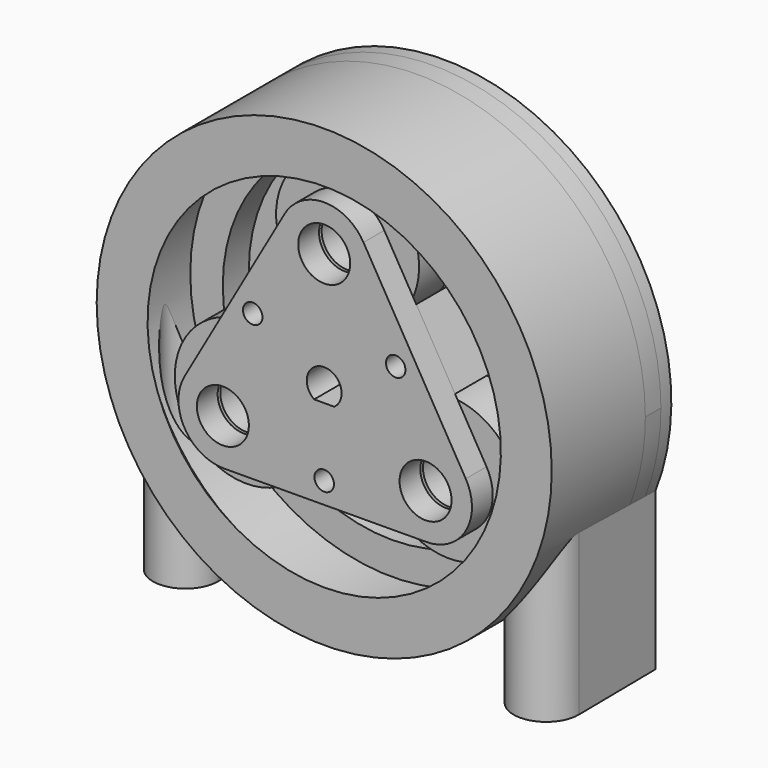
from build123d import *

# Parameters (mm, degrees)
F0_R      = 4
F1_DEPTH  = 4
F3_DEPTH  = 4
F4_R      = 1.5
F5_DEPTH  = 25.4
F7_R      = 35
F7_R_2    = 2.85
F7_R_3    = 4
F8_DEPTH  = 3
F9_R      = 35
F9_R_2    = 1.75
F9_R_3    = 4
F10_DEPTH = 2
F12_R     = 11
F12_R_2   = 4
F13_DEPTH = 7
F15_R     = 35
F15_R_2   = 31
F16_DEPTH = 18
F22_R     = 3.175
F23_DEPTH = 37
F24_R     = 31
F24_R_2   = 26
F25_DEPTH = 5


# Not quite as in the source:
# - after a boolean that leaves OpenCascade's solid faulty, fix() repairs it


with BuildPart() as f1:
    # F0 (on Front) → F1 (new body)
    with BuildSketch(Plane.XZ):
        with BuildLine():
            Line((21.7703811819, -5.3551862172), (6.0422815334, 21.5342373819))
            ThreePointArc((6.0422815334, 21.5342373819), (-0.039598589, 24.9998879957), (-6.0818801224, 21.4656506138))
            Line((-6.0818801224, 21.4656506138), (-21.504754228, -5.5999950346))
            ThreePointArc((-21.504754228, -5.5999950346), (-21.465155639, -12.5998830303), (-15.3832755166, -16.0655336441))
            Line((-15.3832755166, -16.0655336441), (15.7676982376, -15.8893115947))
            ThreePointArc((15.7676982376, -15.8893115947), (21.8099797709, -12.3550742128), (21.7703811819, -5.3551862172))
        make_face()
        with Locations((-15.5884572681, -9)):
            Circle(F0_R, mode=Mode.SUBTRACT)
        with Locations((15.5884572681, -9)):
            Circle(F0_R, mode=Mode.SUBTRACT)
        with Locations((0, 18)):
            Circle(F0_R, mode=Mode.SUBTRACT)
    extrude(amount=F1_DEPTH)

    # F2 (on face) → F3 (join)
    with BuildSketch(Plane.XZ.offset(4)):
        with BuildLine():
            ThreePointArc((-16.6300065653, 2.9547135081), (-5.1558488531, -3.0703556887), (-5.8500069609, -16.0116036406))
            Line((-5.8500069609, -16.0116036406), (5.8028816925, -15.9456828789))
            ThreePointArc((5.8028816925, -15.9456828789), (5.2509372213, -2.906094907), (16.9270942552, 2.9251017194))
            Line((16.9270942552, 2.9251017194), (10.9633508087, 13.1209694563))
            ThreePointArc((10.9633508087, 13.1209694563), (0.0678832955, 6.0001920074), (-10.9074492372, 12.9972456448))
            Line((-10.9074492372, 12.9972456448), (-16.6300065653, 2.9547135081))
        make_face()
        with BuildLine():
            ThreePointArc((-1.5447653543, -2.19), (0, 2.68), (1.5447653543, -2.19))
            Line((1.5447653543, -2.19), (-1.5447653543, -2.19))
        make_face(mode=Mode.SUBTRACT)
    extrude(amount=F3_DEPTH)

    # F4 (on Front) → F5 (cut)
    with BuildSketch(Plane.XZ):
        with Locations((0, -12.7)):
            Circle(F4_R)
        with Locations((10.9985226281, 6.35)):
            Circle(F4_R)
        with Locations((-10.9985226281, 6.35)):
            Circle(F4_R)
        with BuildLine():
            Line((-1.5447653543, -2.19), (1.5447653543, -2.19))
            ThreePointArc((1.5447653543, -2.19), (0, 2.68), (-1.5447653543, -2.19))
        make_face()
    extrude(amount=F5_DEPTH, mode=Mode.SUBTRACT)

    # F14: F1 across face


with BuildPart() as f8:
    # F7 (on offset) → F8 (new body)
    with BuildSketch(Plane.XZ.offset(-2)):
        Circle(F7_R)
        with Locations((-15.5, -15.5)):
            Circle(F7_R_2, mode=Mode.SUBTRACT)
        with Locations((15.5, -15.5)):
            Circle(F7_R_2, mode=Mode.SUBTRACT)
        with Locations((-15.5, 15.5)):
            Circle(F7_R_2, mode=Mode.SUBTRACT)
        Circle(F7_R_3, mode=Mode.SUBTRACT)
        with Locations((15.5, 15.5)):
            Circle(F7_R_2, mode=Mode.SUBTRACT)
    extrude(amount=-F8_DEPTH)

    # F9 (on face) → F10 (join)
    with BuildSketch(Plane(origin=(0, 5, 0), x_dir=(-1, 0, 0), z_dir=(0, 1, 0))):
        Circle(F9_R)
        with Locations((-15.5, -15.5)):
            Circle(F9_R_2, mode=Mode.SUBTRACT)
        with Locations((15.5, -15.5)):
            Circle(F9_R_2, mode=Mode.SUBTRACT)
        with Locations((-15.5, 15.5)):
            Circle(F9_R_2, mode=Mode.SUBTRACT)
        Circle(F9_R_3, mode=Mode.SUBTRACT)
        with Locations((15.5, 15.5)):
            Circle(F9_R_2, mode=Mode.SUBTRACT)
    extrude(amount=F10_DEPTH)

    # F15 (on face) → F16 (join)
    with BuildSketch(Plane.XZ.offset(-2)):
        Circle(F15_R)
        Circle(F15_R_2, mode=Mode.SUBTRACT)
    extrude(amount=F16_DEPTH)

    add(f8.part.fix(), mode=Mode.REPLACE)

    # F17 (on Right) → F18 (revolve)
    with BuildSketch(Plane.YZ):
        Polygon((-16, -32.175), (-11, -32.175), (-16, -27.175), align=None)
    revolve(axis=Axis((0, -8.0179562792, 0), (0, -1, 0)))

    # F20 (on offset) → F21 (join, up to the next surface of F8)
    with BuildSketch(Plane.XY.offset(-37)):
        with BuildLine():
            Line((-32.5682681475, 7), (-32.7496315906, -7.9393043761))
            ThreePointArc((-32.7496315906, -7.9393043761), (-27.7619081825, -12.9999858195), (-22.7501360182, -7.9631196072))
            Line((-22.7501360182, -7.9631196072), (-22.7501360182, 7))
            Line((-22.7501360182, 7), (-32.5682681475, 7))
        make_face()
        with BuildLine():
            ThreePointArc((22.7501360182, -7.9631196072), (27.7619081825, -12.9999858195), (32.7496315906, -7.9393043761))
            Line((32.7496315906, -7.9393043761), (32.5682681475, 7))
            Line((32.5682681475, 7), (22.7501360182, 7))
            Line((22.7501360182, 7), (22.7501360182, -7.9631196072))
        make_face()
    extrude(until=Until.NEXT)

    # F22 (on face) → F23 (cut)
    with BuildSketch(Plane(origin=(0, 0, -37), x_dir=(1, 0, 0), z_dir=(0, 0, -1))):
        with Locations((27.75, 8)):
            Circle(F22_R)
        with Locations((-27.75, 8)):
            Circle(F22_R)
    extrude(amount=-F23_DEPTH, mode=Mode.SUBTRACT)

    # F24 (on face) → F25 (join)
    with BuildSketch(Plane.XZ.offset(-2)):
        Circle(F24_R)
        Circle(F24_R_2, mode=Mode.SUBTRACT)
    extrude(amount=F25_DEPTH)


with BuildPart() as f13:
    # F12 (on offset) → F13 (new body)
    with BuildSketch(Plane.XZ.offset(4.5)):
        with Locations((0, 18)):
            Circle(F12_R)
        with Locations((0, 18)):
            Circle(F12_R_2, mode=Mode.SUBTRACT)
    extrude(amount=F13_DEPTH)


with BuildPart() as f13b:
    # F12 (on offset) → F13, piece 2 (new body)
    with BuildSketch(Plane.XZ.offset(4.5)):
        with Locations((-15.5884572681, -9)):
            Circle(F12_R)
        with Locations((-15.5884572681, -9)):
            Circle(F12_R_2, mode=Mode.SUBTRACT)
    extrude(amount=F13_DEPTH)


with BuildPart() as f13c:
    # F12 (on offset) → F13, piece 3 (new body)
    with BuildSketch(Plane.XZ.offset(4.5)):
        with Locations((15.5884572681, -9)):
            Circle(F12_R)
        with Locations((15.5884572681, -9)):
            Circle(F12_R_2, mode=Mode.SUBTRACT)
    extrude(amount=F13_DEPTH)


with BuildPart() as f1_1:
    add(f1.part)
    add(f1.part.mirror(Plane(origin=(0.0858513894, -8, 0.0050053506), x_dir=(1, 0, 0), z_dir=(0, -1, 0))))


solid = Compound([f8.part, f13.part, f13b.part, f13c.part, f1_1.part])
